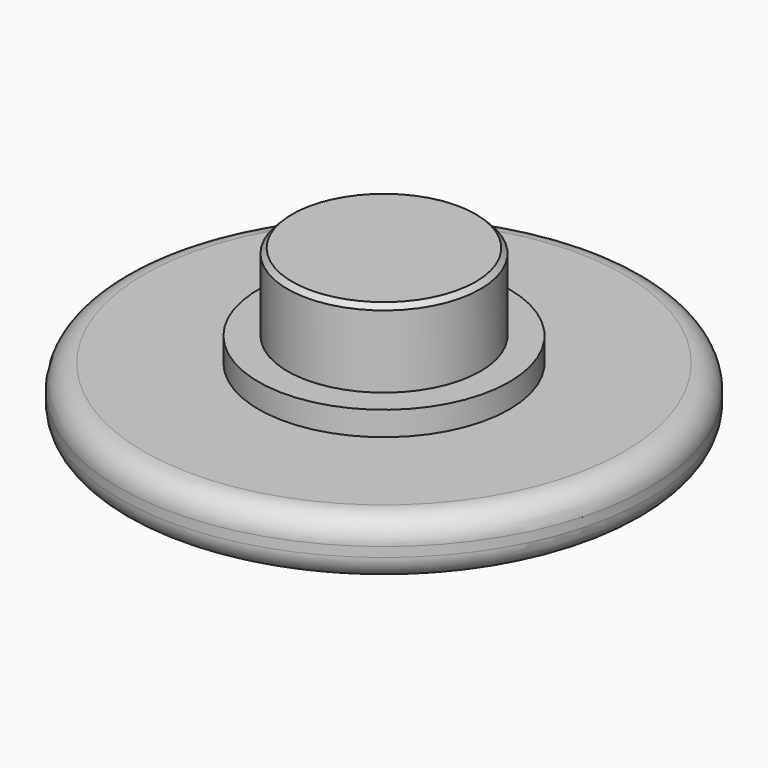
from build123d import *

# Parameters (mm, degrees)
F0_R     = 10.95
F1_DEPTH = 2.4
F2_R     = 4
F3_DEPTH = 4.2
F4_R     = 1
F5_R     = 5.2
F5_R_2   = 4
F6_DEPTH = 1
F7_R     = 1
F8_R     = 8.5
F9_DEPTH = 2
F11_SIZE = 0.2
F12_R    = 3


# Not quite as in the source:
# - a fillet or chamfer that OpenCascade refuses, or shapes differently, is made with other operations: its cross-section is extruded or revolved along the edge and cut away or added


with BuildPart() as f1:
    # F0 (on Top) → F1 (new body)
    with BuildSketch(Plane.XY):
        Circle(F0_R)
    extrude(amount=F1_DEPTH)

    # F2 (on face) → F3 (join)
    with BuildSketch(Plane.XY.offset(2.4)):
        Circle(F2_R)
    extrude(amount=F3_DEPTH)

    # F4
    f4_edges = [f1.edges().sort_by_distance(p)[0] for p in [
        (-10.95, 0, 2.4),
    ]]
    fillet(f4_edges, radius=F4_R)

    # F5 (on face) → F6 (join)
    with BuildSketch(Plane.XY.offset(2.4)):
        Circle(F5_R)
        Circle(F5_R_2, mode=Mode.SUBTRACT)
    extrude(amount=F6_DEPTH)

    # F7
    f7_edges = [f1.edges().sort_by_distance(p)[0] for p in [
        (-10.95, 0, 0),
    ]]
    fillet(f7_edges, radius=F7_R)

    # F8 (on face) → F9 (cut)
    with BuildSketch(Plane(origin=(0, 0, 0), x_dir=(1, 0, 0), z_dir=(0, 0, -1))):
        Circle(F8_R)
    extrude(amount=-F9_DEPTH, mode=Mode.SUBTRACT)

    # F10: fillet of radius 6 on 1 edges, made by hand

    # F10_s1 → F10_t2 (revolve)
    with BuildSketch(Plane.XZ):
        with BuildLine():
            ThreePointArc((8.5, 0), (6.4773537878, 1.4772255751), (4.027864045, 2))
            Line((4.027864045, 2), (8.5, 2))
            Line((8.5, 2), (8.5, 0))
        make_face()
    revolve(axis=Axis((0, 0, 2), (0, 0, -1)))

    # F11
    f11_edges = [f1.edges().sort_by_distance(p)[0] for p in [
        (-4, 0, 6.6),
    ]]
    chamfer(f11_edges, length=F11_SIZE)

    # F12
    f12_edges = [f1.edges().sort_by_distance(p)[0] for p in [
        (-8.5, 0, 0),
    ]]
    fillet(f12_edges, radius=F12_R)


solid = f1.part
